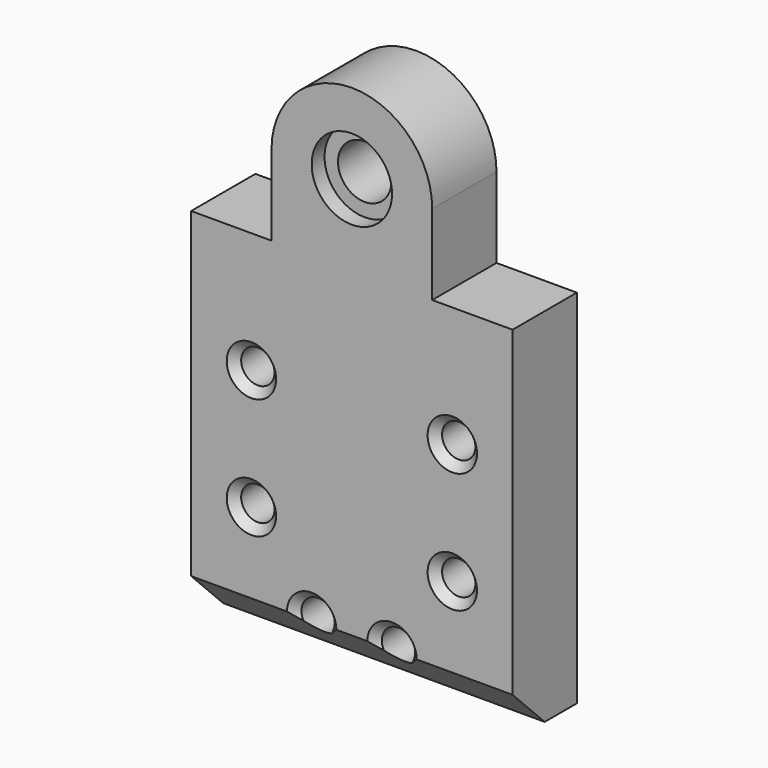
from build123d import *

# Parameters (mm, degrees)
F0_W         = 40
F0_H         = 40
F0_R         = 2.074
F1_DEPTH     = 10
F2_W         = 10
F2_H         = 5
F3_DEPTH     = 10
F4_SIZE      = 1
F5_R         = 3.3235
F6_DEPTH     = 10.001
F7_R         = 5
F7_R_2       = 3.3235
F8_DEPTH     = 2
F10_R        = 3.5
F11_DEPTH    = 5
F12_T1_DEPTH = 65.7168298797


# Not quite as in the source:
# - a fillet or chamfer that OpenCascade refuses, or shapes differently, is made with other operations: its cross-section is extruded or revolved along the edge and cut away or added
# - a pattern or mirror of a feature is missing from the dataset's text; its kind, count and spacing are read off the source's solid


with BuildPart() as f1:
    # F0 (on Front) → F1 (new body)
    with BuildSketch(Plane.XZ):
        Rectangle(F0_W, F0_H)
        with Locations((-5, -15)):
            Circle(F0_R, mode=Mode.SUBTRACT)
        with Locations((-12.5, -5)):
            Circle(F0_R, mode=Mode.SUBTRACT)
        with Locations((5, -15)):
            Circle(F0_R, mode=Mode.SUBTRACT)
        with Locations((12.5, -5)):
            Circle(F0_R, mode=Mode.SUBTRACT)
        with Locations((-12.5, 10)):
            Circle(F0_R, mode=Mode.SUBTRACT)
        with Locations((12.5, 10)):
            Circle(F0_R, mode=Mode.SUBTRACT)
    extrude(amount=F1_DEPTH)

    # F2 (on face) → F3 (join, through all)
    with BuildSketch(Plane.XZ.offset(10)):
        with BuildLine():
            Line((10, 25), (10, 35))
            ThreePointArc((10, 35), (0, 45), (-10, 35))
            Line((-10, 35), (-10, 25))
            Line((-10, 25), (-10, 20))
            Line((-10, 20), (10, 20))
            Line((10, 20), (10, 25))
        make_face()
        with Locations((-15, 22.5)):
            Rectangle(F2_W, F2_H)
        with Locations((15, 22.5)):
            Rectangle(F2_W, F2_H)
    extrude(amount=-F3_DEPTH)

    # F4
    f4_edges = [f1.edges().sort_by_distance(p)[0] for p in [
        (-7.074, -10, -15),
        (2.926, -10, -15),
        (-14.574, -10, 10),
        (-14.574, -10, -5),
        (10.426, -10, -5),
        (10.426, -10, 10),
    ]]
    chamfer(f4_edges, length=F4_SIZE)

    # F5 (on face) → F6 (cut, through all)
    with BuildSketch(Plane.XZ.offset(10)):
        with Locations((0, 35)):
            Circle(F5_R)
    extrude(amount=-F6_DEPTH, mode=Mode.SUBTRACT)

    # F7 (on face) → F8 (cut)
    with BuildSketch(Plane.XZ.offset(10)):
        with Locations((0, 35)):
            Circle(F7_R)
        with Locations((0, 35)):
            Circle(F7_R_2, mode=Mode.SUBTRACT)
    f8 = extrude(amount=-F8_DEPTH, mode=Mode.SUBTRACT)

    # F8_copies: F8 across plane
    add(f8.mirror(Plane.ZX.offset(-5)), mode=Mode.SUBTRACT)

    # F10 (on face) → F11 (cut)
    with BuildSketch(Plane(origin=(0, 0, 0), x_dir=(-1, 0, 0), z_dir=(0, 1, 0))):
        with Locations((0, 10.311)):
            Circle(F10_R)
    extrude(amount=-F11_DEPTH, mode=Mode.SUBTRACT)

    # F12: chamfer of 5 on 1 edges, made by hand

    # F12_s2 → F12_t1 (cut)
    with BuildSketch(Plane.YZ.offset(-32.8584149398)):
        Polygon((-10, -15), (-5, -20), (-10, -20), align=None)
    extrude(amount=F12_T1_DEPTH, mode=Mode.SUBTRACT)


solid = f1.part
